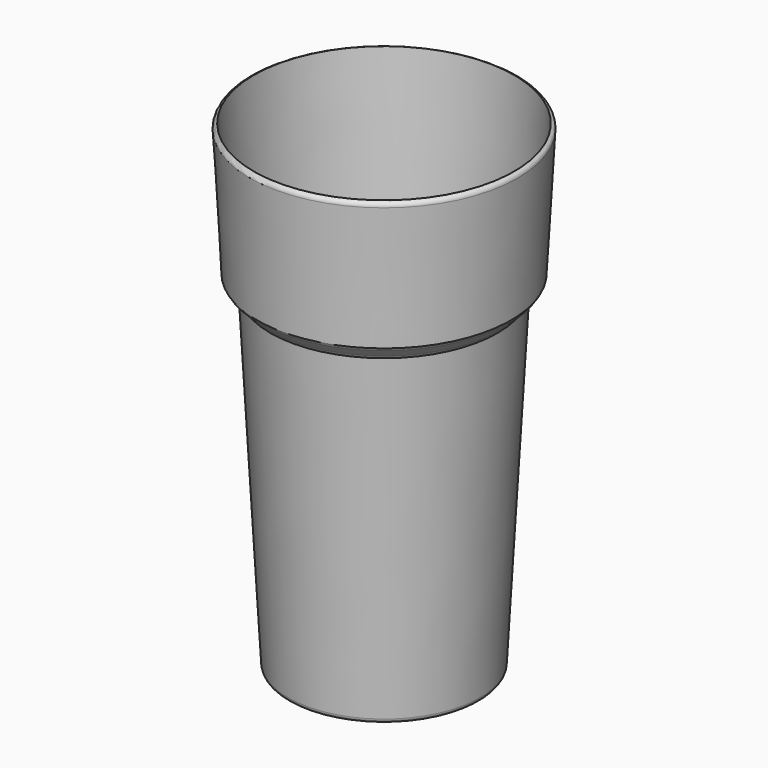
from build123d import *

# Parameters (mm, degrees)
F3_C1_SIZE2 = 0.25
F3_C1_SIZE  = 0.5
F3_C2_SIZE2 = 0.25
F3_C2_SIZE  = 0.5


# Not quite as in the source:
# - a fillet or chamfer that OpenCascade refuses, or shapes differently, is made with other operations: its cross-section is extruded or revolved along the edge and cut away or added


with BuildPart() as f1:
    # F0 (on Front) → F1 (revolve)
    with BuildSketch(Plane.XZ):
        Polygon((-24.2239079518, 85.7203521749), (-25.0227362253, 85.6770823112), (-23.5166698694, 57.8727796674), (-20.7616358603, 55.1226193476), (-17.0000027865, -14.3229160458), (2.9999972135, -14.3229160458), (2.9999972135, -13.5229167386), (-16.2421640236, -13.5229167386), (-19.9793957734, 55.4721326625), (-22.7344297825, 58.2222929823), align=None)
    revolve(axis=Axis((2.9999972135, 0, 16.662178661), (0, 0, -1)))

    # F2: fillet of radius 1 on 2 edges, made by hand

    # F2_s1 → F2_t2 (revolve, cut)
    with BuildSketch(Plane.XZ):
        with BuildLine():
            ThreePointArc((-24.2239458394, 85.7204973112), (-24.7789966166, 85.342605366), (-24.9698980485, 84.6988349638))
            Line((-24.9698980485, 84.6988349638), (-24.9898687726, 84.6977532163))
            ThreePointArc((-24.9898687726, 84.6977532163), (-25.0162129708, 85.1868809465), (-25.0427069494, 85.6760005637))
            Line((-25.0427069494, 85.6760005637), (-25.0238179728, 85.6970530353))
            ThreePointArc((-25.0238179728, 85.6970530353), (-24.6244188052, 85.7186871564), (-24.2289975194, 85.7398488106))
            Line((-24.2289975194, 85.7398488106), (-24.2239458394, 85.7204973112))
        make_face()
    revolve(axis=Axis((2.9999972135, 0, 85.6770823112), (0, 0, -1)), mode=Mode.SUBTRACT)

    # F2_s3 → F2_t4 (revolve, cut)
    with BuildSketch(Plane.XZ):
        with BuildLine():
            ThreePointArc((-17.0513818139, -13.3771534223), (-16.7405637995, -14.0490437922), (-16.0528456074, -14.3230660458))
            Line((-16.0528456074, -14.3230660458), (-16.0528456074, -14.3430660458))
            ThreePointArc((-16.0528456074, -14.3430660458), (-16.526424197, -14.3429160458), (-17.0000027865, -14.3429160458))
            Line((-17.0000027865, -14.3429160458), (-17.0199735106, -14.3239977933))
            ThreePointArc((-17.0199735106, -14.3239977933), (-17.0455881341, -13.851112425), (-17.071352538, -13.3782351698))
            Line((-17.071352538, -13.3782351698), (-17.0513818139, -13.3771534223))
        make_face()
    revolve(axis=Axis((2.9999972135, 0, -14.3229160458), (0, 0, -1)), mode=Mode.SUBTRACT)

    # F3: chamfer of 0.25 x 0.5 on 3 edges, made by hand

    # F3_c1
    f3_c1_edges = [f1.edges().sort_by_distance(p)[0] for p in [
        (26.7616302873, 0, 55.1226193476),
    ]]
    f3_c1_side = f1.faces().sort_by_distance((26.7651689498, 0, 55.1261517501))[0]
    chamfer(f3_c1_edges, length=F3_C1_SIZE, length2=F3_C1_SIZE2, reference=f3_c1_side)

    # F3_c2
    f3_c2_edges = [f1.edges().sort_by_distance(p)[0] for p in [
        (29.5166642964, 0, 57.8727796674),
    ]]
    f3_c2_side = f1.faces().sort_by_distance((29.5131256339, 0, 57.8692472648))[0]
    chamfer(f3_c2_edges, length=F3_C2_SIZE, length2=F3_C2_SIZE2, reference=f3_c2_side)


solid = f1.part
